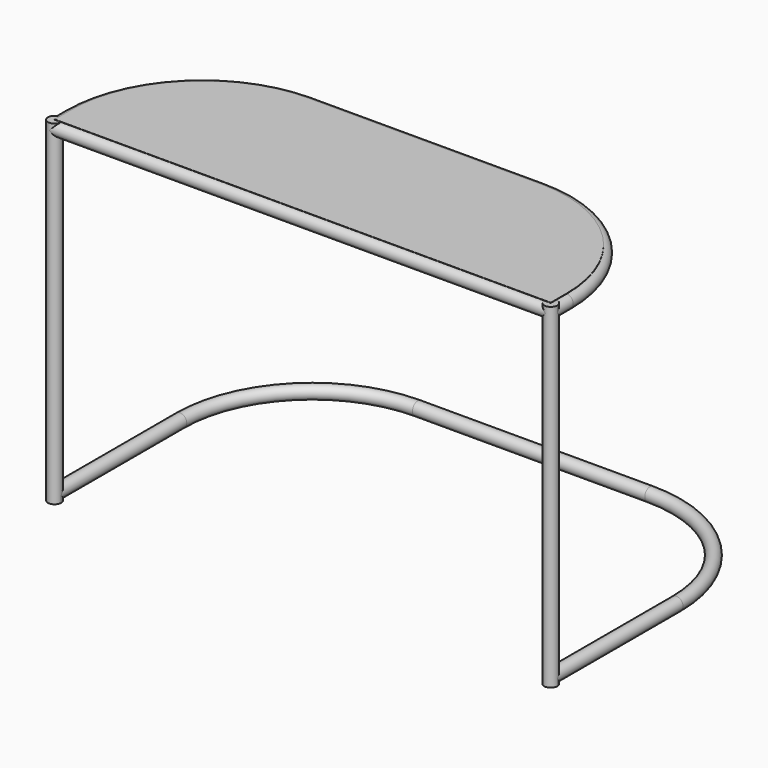
from build123d import *
from build123d import SkipClean  # not in build123d's __all__

# Parameters (mm, degrees)
F0_R      = 2.5
F1_DEPTH  = 127
F5_R      = 2.5
F7_R      = 2.5
F11_R     = 2.5
F20_DEPTH = 0.1


# Not quite as in the source:
# - the program builds the solid bodies; features that only make, move or delete a surface that nothing else refers to are left out


with BuildPart() as f1:
    # F0 (on Top) → F1 (new body)
    with BuildSketch(Plane.XY):
        with Locations((94, 0)):
            Circle(F0_R)
    extrude(amount=F1_DEPTH)



with BuildPart() as f1b:
    # F0 (on Top) → F1, piece 2 (new body)
    with BuildSketch(Plane.XY):
        with Locations((-94, 0)):
            Circle(F0_R)
    extrude(amount=F1_DEPTH)


with BuildPart() as f1_1:
    add(f1.part, clean=False)

    add(f1b.part)  # F6 merges F1b
    # F6: sweep along a path in F3
    with BuildLine(Plane.XY.offset(124.5)) as f6_path:
        Line((-94, 0), (94, 0))
    # F5 (on offset) → F6 (sweep)
    with BuildSketch(Plane.YZ.offset(94)):
        with Locations((0, 124.5)):
            Circle(F5_R)
    sweep(path=f6_path.line)

    # F9: sweep along a path in F8
    with BuildLine(Plane.XY) as f9_path:
        Line((94, 0), (94, 59.5))
        ThreePointArc((94, 59.5), (79.3553390593, 94.8553390593), (44, 109.5))
        Line((44, 109.5), (-44, 109.5))
        ThreePointArc((-44, 109.5), (-79.3553390593, 94.8553390593), (-94, 59.5))
        Line((-94, 59.5), (-94, 0))
    # F7 (on Front) → F9 (sweep)
    with BuildSketch(Plane.XZ):
        with Locations((94, 2.5)):
            Circle(F7_R)
    sweep(path=f9_path.line)

    # F12: sweep along a path in F10
    with BuildLine(Plane.XY.offset(124.5)) as f12_path:
        Line((94, 0), (94, 7.5))
        ThreePointArc((94, 7.5), (79.3553390593, 42.8553390593), (44, 57.5))
        Line((44, 57.5), (-44, 57.5))
        ThreePointArc((-44, 57.5), (-79.3553390593, 42.8553390593), (-94, 7.5))
        Line((-94, 7.5), (-94, 0))
    # F11 (on Front) → F12 (sweep)
    with BuildSketch(Plane.XZ):
        with Locations((94, 124.5)):
            Circle(F11_R)
    with SkipClean():  # cleaning this boolean's faces spoils the solid; the shape is the same uncleaned
        sweep(path=f12_path.line)


with BuildPart() as f20:
    # F19 (on offset) → F20 (new body)
    with BuildSketch(Plane.XY.offset(127)):
        with BuildLine():
            Line((-94, 7.5), (-94, 0))
            Line((-94, 0), (94, 0))
            Line((94, 0), (94, 7.5))
            ThreePointArc((94, 7.5), (79.3553390593, 42.8553390593), (44, 57.5))
            Line((44, 57.5), (-44, 57.5))
            ThreePointArc((-44, 57.5), (-79.3553390593, 42.8553390593), (-94, 7.5))
        make_face()
    extrude(amount=F20_DEPTH)


solid = Compound([f1_1.part, f20.part])
